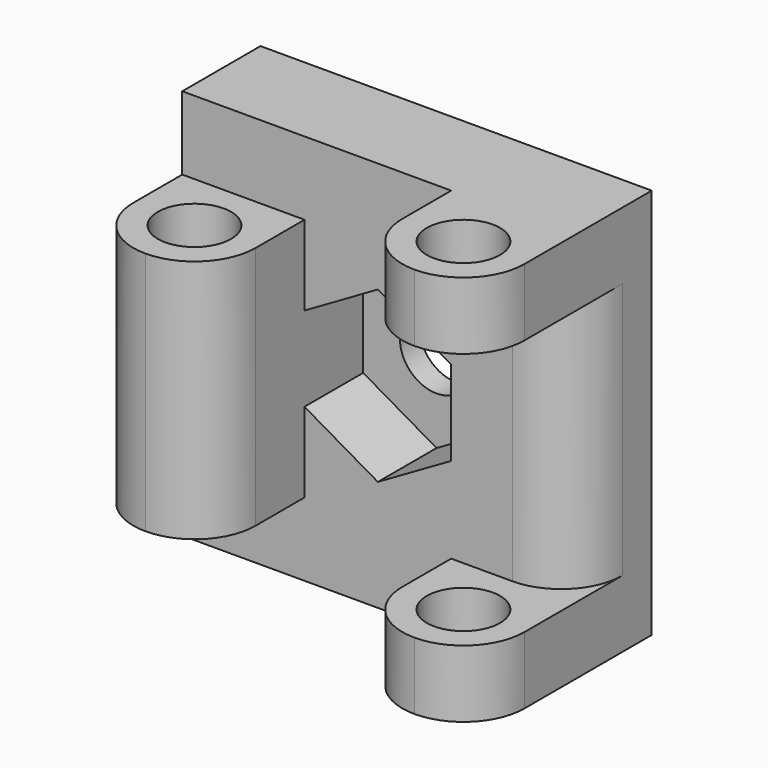
from build123d import *

# Parameters (mm, degrees)
F0_W      = 32
F0_H      = 32
F1_DEPTH  = 8
F2_W      = 10
F2_H      = 20
F2_H_2    = 5.5
F3_DEPTH  = 10
F5_DEPTH  = 6
F6_R      = 3
F7_DEPTH  = 25
F8_R      = 3
F9_DEPTH  = 25
F10_R     = 3
F11_DEPTH = 32.001
F12_R     = 4.99999
F13_R     = 4.99999
F14_R     = 5


# Not quite as in the source:
# - a fillet or chamfer is up to 0.001 mm smaller than in the source, because OpenCascade refuses the exact size


with BuildPart() as f1:
    # F0 (on Front) → F1 (new body)
    with BuildSketch(Plane.XZ):
        Rectangle(F0_W, F0_H)
    extrude(amount=F1_DEPTH)

    # F2 (on face) → F3 (join)
    with BuildSketch(Plane.XZ.offset(8)):
        with Locations((-11, 0)):
            Rectangle(F2_W, F2_H)
        with Locations((11, -13.25)):
            Rectangle(F2_W, F2_H_2)
        with Locations((11, 13.25)):
            Rectangle(F2_W, F2_H_2)
    extrude(amount=F3_DEPTH)

    # F4 (on face) → F5 (cut)
    with BuildSketch(Plane.XZ.offset(8)):
        Polygon((6, -3.4641016151), (6, 3.4641016151), (0, 6.9282032303), (-6, 3.4641016151), (-6, -3.4641016151), (0, -6.9282032303), align=None)
    extrude(amount=-F5_DEPTH, mode=Mode.SUBTRACT)

    # F6 (on face) → F7 (cut)
    with BuildSketch(Plane(origin=(0, 0, 0), x_dir=(-1, 0, 0), z_dir=(0, 1, 0))):
        Circle(F6_R)
    extrude(amount=-F7_DEPTH, mode=Mode.SUBTRACT)

    # F8 (on face) → F9 (cut)
    with BuildSketch(Plane(origin=(0, 0, -10), x_dir=(1, 0, 0), z_dir=(0, 0, -1))):
        with Locations((-11, 13)):
            Circle(F8_R)
    extrude(amount=-F9_DEPTH, mode=Mode.SUBTRACT)

    # F10 (on face) → F11 (cut, through all)
    with BuildSketch(Plane(origin=(0, 0, -16), x_dir=(1, 0, 0), z_dir=(0, 0, -1))):
        with Locations((11, 13)):
            Circle(F10_R)
    extrude(amount=-F11_DEPTH, mode=Mode.SUBTRACT)

    # F12 (radius 5 in the source; OpenCascade refuses exactly that, so slightly less here)
    f12_edges = [f1.edges().sort_by_distance(p)[0] for p in [
        (6, -18, 13.25),
        (16, -18, 13.25),
        (16, -18, -13.25),
        (6, -18, -13.25),
    ]]
    fillet(f12_edges, radius=F12_R)

    # F13 (radius 5 in the source; OpenCascade refuses exactly that, so slightly less here)
    f13_edges = [f1.edges().sort_by_distance(p)[0] for p in [
        (-6, -18, 0),
        (-16, -18, 0),
    ]]
    fillet(f13_edges, radius=F13_R)

    # F14
    f14_edges = [f1.edges().sort_by_distance(p)[0] for p in [
        (16, -8, 0),
    ]]
    fillet(f14_edges, radius=F14_R)


solid = f1.part
